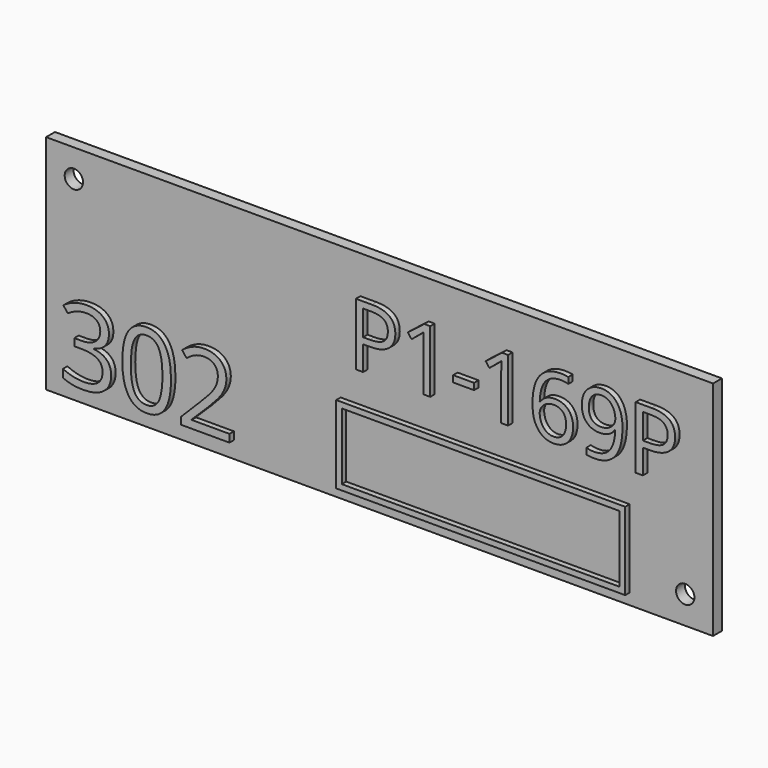
from build123d import *

# Parameters (mm, degrees)
F0_W         = 120
F0_H         = 40
F1_DEPTH     = 2
F3_D         = 3.3
F4_TEXT_SIZE = 15.681149951
F5_DEPTH     = 1
F6_TEXT_SIZE = 18.5356140827
F7_DEPTH     = 1
F8_W         = 52
F8_H         = 14
F8_W_2       = 49.99999962
F8_H_2       = 11.99999962
F9_DEPTH     = 1


# Not quite as in the source:
# - Text() gives the source's letters only with a copy of the font that has no kerning and outlines rounded to 1/6400 em; it was checked with that copy


with BuildPart() as f1:
    # F0 (on Front) → F1 (new body)
    with BuildSketch(Plane.XZ):
        Rectangle(F0_W, F0_H)
    extrude(amount=F1_DEPTH)

    # F3 (through all)
    with Locations(Plane.XZ.offset(2)):
        with Locations((-55, 15), (55, -15)):
            Hole(F3_D / 2)

    # F4 (on face) → F5 (join)
    with BuildSketch(Plane.XZ.offset(2)):
        with Locations((-5, 2)):
            Text('P1-169P', F4_TEXT_SIZE, font='Open Sans', text_align=(TextAlign.LEFT, TextAlign.BOTTOM))
    extrude(amount=F5_DEPTH)

    # F6 (on face) → F7 (join)
    with BuildSketch(Plane.XZ.offset(2)):
        with Locations((-57, -17)):
            Text('302', F6_TEXT_SIZE, font='Open Sans', text_align=(TextAlign.LEFT, TextAlign.BOTTOM))
    extrude(amount=F7_DEPTH)

    # F8 (on face) → F9 (join)
    with BuildSketch(Plane.XZ.offset(2)):
        with Locations((19, -11)):
            Rectangle(F8_W, F8_H)
        with Locations((19, -11)):
            Rectangle(F8_W_2, F8_H_2, mode=Mode.SUBTRACT)
    extrude(amount=F9_DEPTH)


solid = f1.part
